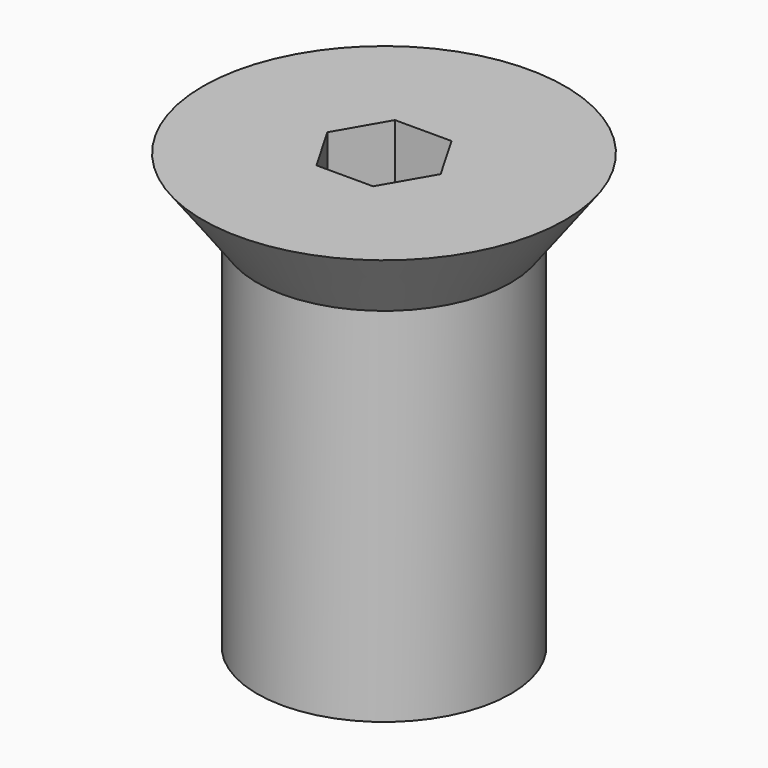
from build123d import *

# Parameters (mm, degrees)
F3_DEPTH = 0.254


# Not quite as in the source:
# - a feature names something its author has since deleted; it is built from what else it names


with BuildPart() as f1:
    # F0 (on Front) → F1 (revolve)
    with BuildSketch(Plane.XZ):
        Polygon((-45.2334927974, 40.7203510404), (-45.8684927974, 40.7203510404), (-45.6779927974, 40.4649959532), (-45.6779927974, 39.1963510404), (-45.2334927974, 39.1963510404), align=None)
    revolve(axis=Axis((-45.2334927974, 0, 39.9583510404), (0, 0, -1)))

    # F2 (on face) → F3 (cut)
    with BuildSketch(Plane.XY.offset(40.7203510404)):
        Polygon((-45.1342007585, 0.1719788561), (-45.3327848362, 0.1719788561), (-45.4320768751, 0), (-45.3327848362, -0.1719788561), (-45.1342007585, -0.1719788561), (-45.0349087197, 0), align=None)
    extrude(amount=-F3_DEPTH, mode=Mode.SUBTRACT)


solid = f1.part
